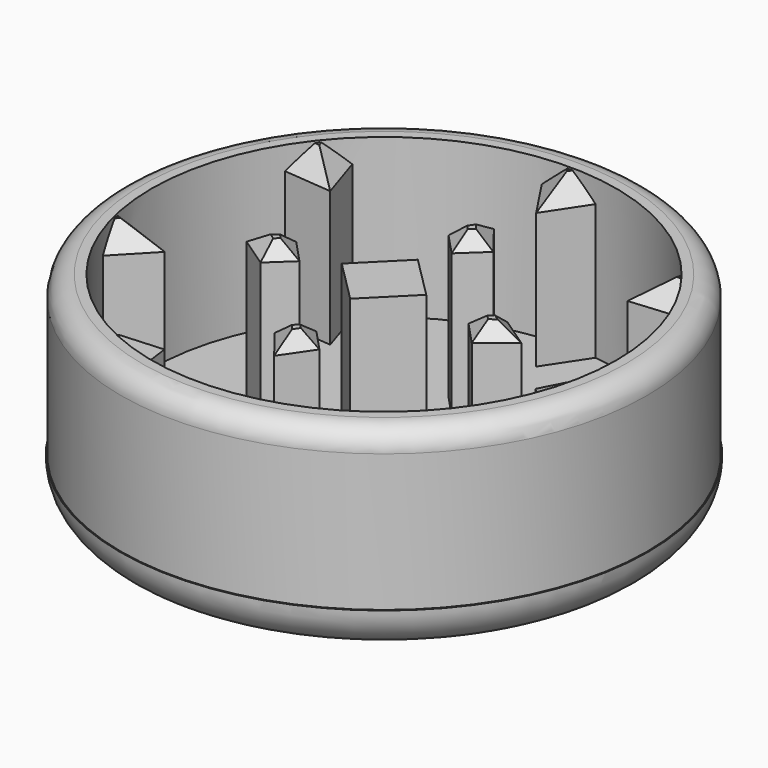
from build123d import *

# Parameters (mm, degrees)
F0_R      = 25
F1_DEPTH  = 4
F3_DEPTH  = 14.8
F4_R      = 24.9
F4_R_2    = 22
F5_DEPTH  = 15
F6_SIZE   = 1.3
F7_SIZE   = 2
F8_R      = 3.99999
F9_R      = 2
F10_R     = 4.5599564507
F11_DEPTH = 0.2


# Not quite as in the source:
# - a fillet or chamfer is up to 0.001 mm smaller than in the source, because OpenCascade refuses the exact size
# - a feature names something its author has since deleted; it is built from what else it names


with BuildPart() as f1:
    # F0 (on Top) → F1 (new body)
    with BuildSketch(Plane.XY):
        Circle(F0_R)
    extrude(amount=F1_DEPTH)

    # F2 (on face) → F3 (join)
    with BuildSketch(Plane.XY.offset(4)):
        Polygon((1.9764285987, -10.1112626395), (0, -8), (-2.2552952007, -10.1112626395), (0, -13), align=None)
        Polygon((0, -4), (4, 0), (0, 4), (-4, 0), align=None)
        Polygon((-10.1112626395, -1.9764285987), (-8, 0), (-10.1112626395, 2.2552952007), (-13, 0), align=None)
        Polygon((-1.9764285987, 10.1112626395), (0, 8), (2.2552952007, 10.1112626395), (0, 13), align=None)
        Polygon((10.1112626395, 1.9764285987), (8, 0), (10.1112626395, -2.2552952007), (13, 0), align=None)
        with BuildLine():
            Line((14.0729666844, 11.2228164335), (18.6727000521, 11.6331540333))
            ThreePointArc((18.6727000521, 11.6331540333), (17.2002926143, 13.7167756409), (15.4965532289, 15.6159161763))
            Line((15.4965532289, 15.6159161763), (14.0729666844, 11.2228164335))
        make_face()
        with BuildLine():
            ThreePointArc((20.7374041193, -7.3457518602), (21.448414068, -4.895460547), (21.8709577964, -2.3793287015))
            Line((21.8709577964, -2.3793287015), (17.5487024193, -4.0053768112))
            Line((17.5487024193, -4.0053768112), (20.7374041193, -7.3457518602))
        make_face()
        with BuildLine():
            ThreePointArc((7.1864199187, -20.793156777), (9.5454422606, -19.8213150939), (11.776085057, -18.5828905376))
            Line((11.776085057, -18.5828905376), (7.8099073041, -16.2174396222))
            Line((7.8099073041, -16.2174396222), (7.1864199187, -20.793156777))
        make_face()
        with BuildLine():
            Line((-7.1864199187, -20.793156777), (-7.8099073041, -16.2174396222))
            Line((-7.8099073041, -16.2174396222), (-11.776085057, -18.5828905376))
            ThreePointArc((-11.776085057, -18.5828905376), (-9.5454422606, -19.8213150939), (-7.1864199187, -20.793156777))
        make_face()
        with BuildLine():
            Line((-20.7374041193, -7.3457518602), (-17.5487024193, -4.0053768112))
            Line((-17.5487024193, -4.0053768112), (-21.8709577964, -2.3793287015))
            ThreePointArc((-21.8709577964, -2.3793287015), (-21.448414068, -4.895460547), (-20.7374041193, -7.3457518602))
        make_face()
        with BuildLine():
            Line((-18.6727000521, 11.6331540333), (-14.0729666844, 11.2228164335))
            Line((-14.0729666844, 11.2228164335), (-15.4965532289, 15.6159161763))
            ThreePointArc((-15.4965532289, 15.6159161763), (-17.2002926143, 13.7167756409), (-18.6727000521, 11.6331540333))
        make_face()
        with BuildLine():
            Line((0, 18), (2.547071992, 21.8520576667))
            ThreePointArc((2.547071992, 21.8520576667), (0, 22), (-2.547071992, 21.8520576667))
            Line((-2.547071992, 21.8520576667), (0, 18))
        make_face()
    extrude(amount=F3_DEPTH)

    # F4 (on face) → F5 (join)
    with BuildSketch(Plane.XY.offset(4)):
        Circle(F4_R)
        Circle(F4_R_2, mode=Mode.SUBTRACT)
    extrude(amount=F5_DEPTH)

    # F6
    f6_edges = [f1.edges().sort_by_distance(p)[0] for p in [
        (-9.055631, -0.988214, 18.8),
        (-9.055631, 1.127648, 18.8),
        (-11.555631, 1.127648, 18.8),
        (-11.555631, -0.988214, 18.8),
        (0.988214, -9.055631, 18.8),
        (-1.127648, -9.055631, 18.8),
        (-1.127648, -11.555631, 18.8),
        (0.988214, -11.555631, 18.8),
        (9.055631, 0.988214, 18.8),
        (9.055631, -1.127648, 18.8),
        (11.555631, -1.127648, 18.8),
        (11.555631, 0.988214, 18.8),
        (-0.988214, 9.055631, 18.8),
        (1.127648, 9.055631, 18.8),
        (1.127648, 11.555631, 18.8),
        (-0.988214, 11.555631, 18.8),
    ]]
    chamfer(f6_edges, length=F6_SIZE)

    # F7
    f7_edges = [f1.edges().sort_by_distance(p)[0] for p in [
        (14.78476, 13.419366, 18.8),
        (16.372833, 11.427985, 18.8),
        (19.70983, -3.192353, 18.8),
        (19.143053, -5.675564, 18.8),
        (9.792996, -17.400165, 18.8),
        (7.498164, -18.505298, 18.8),
        (-9.792996, -17.400165, 18.8),
        (-7.498164, -18.505298, 18.8),
        (-19.143053, -5.675564, 18.8),
        (-19.70983, -3.192353, 18.8),
        (-16.372833, 11.427985, 18.8),
        (-1.273536, 19.926029, 18.8),
        (1.273536, 19.926029, 18.8),
        (-14.78476, 13.419366, 18.8),
    ]]
    chamfer(f7_edges, length=F7_SIZE)

    # F8 (radius 4 in the source; OpenCascade refuses exactly that, so slightly less here)
    f8_edges = [f1.edges().sort_by_distance(p)[0] for p in [
        (-25, 0, 0),
    ]]
    fillet(f8_edges, radius=F8_R)

    # F9
    f9_edges = [f1.edges().sort_by_distance(p)[0] for p in [
        (-24.9, 0, 19),
    ]]
    fillet(f9_edges, radius=F9_R)

    # F10 (on face) → F11 (cut)
    with BuildSketch(Plane.XY.offset(18.8)):
        Circle(F10_R)
    extrude(amount=-F11_DEPTH, mode=Mode.SUBTRACT)


solid = f1.part
